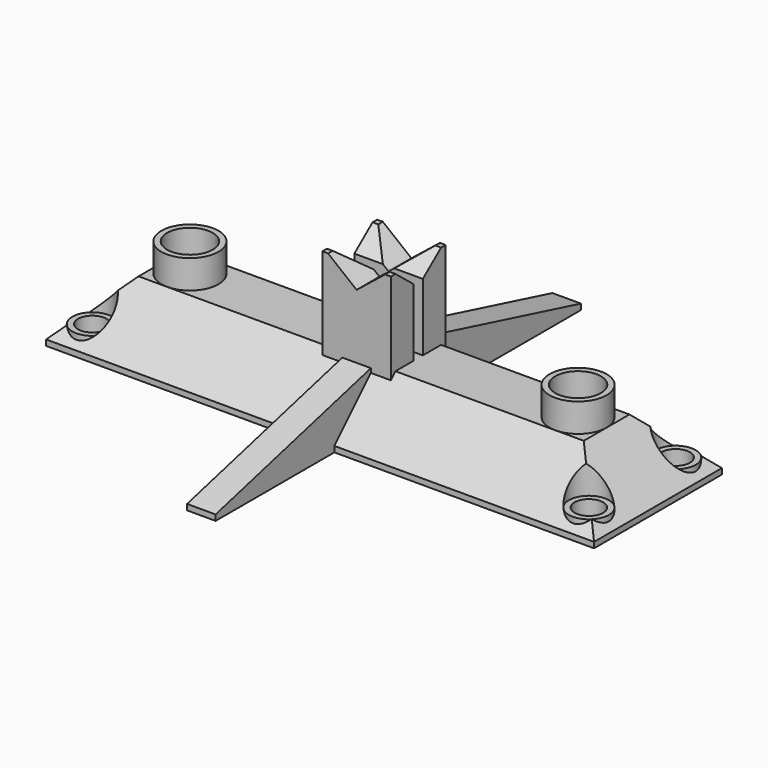
from build123d import *

# Parameters (mm, degrees)
F0_R         = 3.5
F0_R_2       = 5
F0_W         = 5
F0_H         = 26
F0_W_2       = 2.5
F0_H_2       = 6
F0_W_3       = 3.5
F1_DEPTH     = 10
F0_R_3       = 4
F2_DEPTH     = 15
F3_DEPTH     = 1
F4_T4_DEPTH  = 74.2902937834
F4_S5_R      = 5
F4_T6_DEPTH  = 39
F4_T10_DEPTH = 74.2902937834
F4_S11_R     = 5
F4_T12_DEPTH = 39
F4_T16_DEPTH = 91.7902937834
F4_T21_DEPTH = 68.6451468917
F4_S22_R     = 5
F4_T23_DEPTH = 36
F4_T27_DEPTH = 68.6451468917
F4_S28_R     = 5
F4_T29_DEPTH = 36
F4_T33_DEPTH = 91.7902937834
F4_T38_DEPTH = 91.7902937834
F4_T43_DEPTH = 68.6451468917
F4_S44_R     = 5
F4_T45_DEPTH = 36
F4_T49_DEPTH = 68.6451468917
F4_S50_R     = 5
F4_T51_DEPTH = 36
F4_T55_DEPTH = 91.7902937834
F5_SIZE2     = 9
F5_SIZE      = 35
F0_R_4       = 2.5
F6_DEPTH     = 3
F7_DEPTH     = 25
F8_W         = 2
F8_H         = 7
F10_DEPTH    = 25
F11_DEPTH    = 25


# Not quite as in the source:
# - a fillet or chamfer that OpenCascade refuses, or shapes differently, is made with other operations: its cross-section is extruded or revolved along the edge and cut away or added


with BuildPart() as f1:
    # F0 (on Top) → F1 (new body)
    with BuildSketch(Plane.XY):
        Polygon((-2.5, 14), (-48, 14), (-48, -14), (-2.5, -14), (-2.5, -6), (-6, -6), (-6, 0), (-6, 6), (-2.5, 6), align=None)
        with Locations((-43.5, -9.5)):
            Circle(F0_R, mode=Mode.SUBTRACT)
        with Locations((-43.5, 9.5)):
            Circle(F0_R, mode=Mode.SUBTRACT)
        with Locations((-34, 0)):
            Circle(F0_R_2, mode=Mode.SUBTRACT)
        Polygon((48, 14), (2.5, 14), (2.5, 6), (6, 6), (6, 0), (6, -6), (2.5, -6), (2.5, -14), (48, -14), align=None)
        with Locations((43.5, -9.5)):
            Circle(F0_R, mode=Mode.SUBTRACT)
        with Locations((34, 0)):
            Circle(F0_R_2, mode=Mode.SUBTRACT)
        with Locations((43.5, 9.5)):
            Circle(F0_R, mode=Mode.SUBTRACT)
        Polygon((-2.5, -6), (-2.5, -14), (2.5, -14), (2.5, -6), (0, -6), align=None)
        with Locations((0, -27)):
            Rectangle(F0_W, F0_H)
        Polygon((2.5, 14), (-2.5, 14), (-2.5, 6), (0, 6), (2.5, 6), align=None)
        with Locations((0, 27)):
            Rectangle(F0_W, F0_H)
        with Locations((1.25, -3)):
            Rectangle(F0_W_2, F0_H_2)
        with Locations((4.25, -3)):
            Rectangle(F0_W_3, F0_H_2)
        with Locations((-4.25, -3)):
            Rectangle(F0_W_3, F0_H_2)
        with Locations((-1.25, -3)):
            Rectangle(F0_W_2, F0_H_2)
        with Locations((-1.25, 3)):
            Rectangle(F0_W_2, F0_H_2)
        with Locations((-4.25, 3)):
            Rectangle(F0_W_3, F0_H_2)
        with Locations((4.25, 3)):
            Rectangle(F0_W_3, F0_H_2)
        with Locations((1.25, 3)):
            Rectangle(F0_W_2, F0_H_2)
    extrude(amount=F1_DEPTH)

    # F0 (on Top) → F2 (join)
    with BuildSketch(Plane.XY):
        with Locations((-34, 0)):
            Circle(F0_R_2)
        with Locations((-34, 0)):
            Circle(F0_R_3, mode=Mode.SUBTRACT)
        with Locations((34, 0)):
            Circle(F0_R_2)
        with Locations((34, 0)):
            Circle(F0_R_3, mode=Mode.SUBTRACT)
    extrude(amount=F2_DEPTH)

    # F0 (on Top) → F3 (join)
    with BuildSketch(Plane.XY):
        with Locations((-34, 0)):
            Circle(F0_R_3)
        with Locations((34, 0)):
            Circle(F0_R_3)
    extrude(amount=F3_DEPTH)

    # F4: chamfer of 9 on 6 edges, made by hand


with BuildPart() as f4_tool2:
    # F4_s3 → F4_t4 (new body)
    with BuildSketch(Plane.XZ.offset(37.1451468917)):
        Polygon((39, 10), (48, 1), (48, 10), align=None)
    extrude(amount=-F4_T4_DEPTH)

    # F4_s5 → F4_t6 (cut, symmetric)
    with BuildSketch(Plane.XY.offset(5.5)):
        with Locations((34, 0)):
            Circle(F4_S5_R)
    extrude(amount=F4_T6_DEPTH, both=True, mode=Mode.SUBTRACT)


with BuildPart() as f1_1:
    add(f1.part)

    # F4_t1: cut F4_tool2
    add(f4_tool2.part, mode=Mode.SUBTRACT)


with BuildPart() as f4_tool8:
    # F4_s9 → F4_t10 (new body)
    with BuildSketch(Plane.XZ.offset(-37.1451468917)):
        Polygon((-48, 1), (-39, 10), (-48, 10), align=None)
    extrude(amount=F4_T10_DEPTH)

    # F4_s11 → F4_t12 (cut, symmetric)
    with BuildSketch(Plane.XY.offset(5.5)):
        with Locations((-34, 0)):
            Circle(F4_S11_R)
    extrude(amount=F4_T12_DEPTH, both=True, mode=Mode.SUBTRACT)


with BuildPart() as f1_2:
    add(f1_1.part)

    # F4_t7: cut F4_tool8
    add(f4_tool8.part, mode=Mode.SUBTRACT)


with BuildPart() as f4_tool14:
    # F4_s15 → F4_t16 (new body)
    with BuildSketch(Plane.YZ.offset(20.6451468917)):
        Polygon((14, 1), (5, 10), (14, 10), align=None)
    extrude(amount=-F4_T16_DEPTH)

    split(bisect_by=Plane.YZ.offset(2.5), keep=Keep.TOP)


with BuildPart() as f1_3:
    add(f1_2.part)

    # F4_t13: cut F4_tool14
    add(f4_tool14.part, mode=Mode.SUBTRACT)


with BuildPart() as f4_tool19:
    # F4_s20 → F4_t21 (new body)
    with BuildSketch(Plane.YZ.offset(-2.5)):
        Polygon((14, 1), (5, 10), (14, 10), align=None)
    extrude(amount=-F4_T21_DEPTH)

    # F4_s22 → F4_t23 (cut, symmetric)
    with BuildSketch(Plane.XY.offset(5.5)):
        with Locations((-34, 0)):
            Circle(F4_S22_R)
    extrude(amount=F4_T23_DEPTH, both=True, mode=Mode.SUBTRACT)


with BuildPart() as f1_4:
    add(f1_3.part)

    # F4_t18: cut F4_tool19
    add(f4_tool19.part, mode=Mode.SUBTRACT)


with BuildPart() as f4_tool25:
    # F4_s26 → F4_t27 (new body)
    with BuildSketch(Plane.YZ.offset(71.1451468917)):
        Polygon((5, 10), (14, 1), (14, 10), align=None)
    extrude(amount=-F4_T27_DEPTH)

    # F4_s28 → F4_t29 (cut, symmetric)
    with BuildSketch(Plane.XY.offset(5.5)):
        with Locations((34, 0)):
            Circle(F4_S28_R)
    extrude(amount=F4_T29_DEPTH, both=True, mode=Mode.SUBTRACT)


with BuildPart() as f1_5:
    add(f1_4.part)

    # F4_t24: cut F4_tool25
    add(f4_tool25.part, mode=Mode.SUBTRACT)


with BuildPart() as f4_tool31:
    # F4_s32 → F4_t33 (new body)
    with BuildSketch(Plane.YZ.offset(71.1451468917)):
        Polygon((5, 10), (14, 1), (14, 10), align=None)
    extrude(amount=-F4_T33_DEPTH)

    split(bisect_by=Plane.YZ.offset(-2.5), keep=Keep.BOTTOM)


with BuildPart() as f1_6:
    add(f1_5.part)

    # F4_t30: cut F4_tool31
    add(f4_tool31.part, mode=Mode.SUBTRACT)


with BuildPart() as f4_tool36:
    # F4_s37 → F4_t38 (new body)
    with BuildSketch(Plane.YZ.offset(-20.6451468917)):
        Polygon((-5, 10), (-14, 1), (-14, 10), align=None)
    extrude(amount=F4_T38_DEPTH)

    split(bisect_by=Plane.YZ.offset(-2.5), keep=Keep.BOTTOM)


with BuildPart() as f1_7:
    add(f1_6.part)

    # F4_t35: cut F4_tool36
    add(f4_tool36.part, mode=Mode.SUBTRACT)


with BuildPart() as f4_tool41:
    # F4_s42 → F4_t43 (new body)
    with BuildSketch(Plane.YZ.offset(2.5)):
        Polygon((-5, 10), (-14, 1), (-14, 10), align=None)
    extrude(amount=F4_T43_DEPTH)

    # F4_s44 → F4_t45 (cut, symmetric)
    with BuildSketch(Plane.XY.offset(5.5)):
        with Locations((34, 0)):
            Circle(F4_S44_R)
    extrude(amount=F4_T45_DEPTH, both=True, mode=Mode.SUBTRACT)


with BuildPart() as f1_8:
    add(f1_7.part)

    # F4_t40: cut F4_tool41
    add(f4_tool41.part, mode=Mode.SUBTRACT)


with BuildPart() as f4_tool47:
    # F4_s48 → F4_t49 (new body)
    with BuildSketch(Plane.YZ.offset(-71.1451468917)):
        Polygon((-14, 1), (-5, 10), (-14, 10), align=None)
    extrude(amount=F4_T49_DEPTH)

    # F4_s50 → F4_t51 (cut, symmetric)
    with BuildSketch(Plane.XY.offset(5.5)):
        with Locations((-34, 0)):
            Circle(F4_S50_R)
    extrude(amount=F4_T51_DEPTH, both=True, mode=Mode.SUBTRACT)


with BuildPart() as f1_9:
    add(f1_8.part)

    # F4_t46: cut F4_tool47
    add(f4_tool47.part, mode=Mode.SUBTRACT)


with BuildPart() as f4_tool53:
    # F4_s54 → F4_t55 (new body)
    with BuildSketch(Plane.YZ.offset(-71.1451468917)):
        Polygon((-14, 1), (-5, 10), (-14, 10), align=None)
    extrude(amount=F4_T55_DEPTH)

    split(bisect_by=Plane.YZ.offset(2.5), keep=Keep.TOP)


with BuildPart() as f1_10:
    add(f1_9.part)

    # F4_t52: cut F4_tool53
    add(f4_tool53.part, mode=Mode.SUBTRACT)

    # F5
    f5_edges = [f1_10.edges().sort_by_distance(p)[0] for p in [
        (0, 40, 10),
        (0, -40, 10),
    ]]
    f5_side = f1_10.faces().sort_by_distance((0, 0, 10))[0]
    chamfer(f5_edges, length=F5_SIZE, length2=F5_SIZE2, reference=f5_side)

    # F0 (on Top) → F6 (join)
    with BuildSketch(Plane.XY):
        with Locations((-43.5, -9.5)):
            Circle(F0_R)
        with Locations((-43.5, -9.5)):
            Circle(F0_R_4, mode=Mode.SUBTRACT)
        with Locations((-43.5, 9.5)):
            Circle(F0_R)
        with Locations((-43.5, 9.5)):
            Circle(F0_R_4, mode=Mode.SUBTRACT)
        with Locations((43.5, 9.5)):
            Circle(F0_R)
        with Locations((43.5, 9.5)):
            Circle(F0_R_4, mode=Mode.SUBTRACT)
        with Locations((43.5, -9.5)):
            Circle(F0_R)
        with Locations((43.5, -9.5)):
            Circle(F0_R_4, mode=Mode.SUBTRACT)
    extrude(amount=F6_DEPTH)

    # F0 (on Top) → F7 (join)
    with BuildSketch(Plane.XY):
        with Locations((4.25, -3)):
            Rectangle(F0_W_3, F0_H_2)
        with Locations((1.25, -3)):
            Rectangle(F0_W_2, F0_H_2)
        with Locations((-1.25, -3)):
            Rectangle(F0_W_2, F0_H_2)
        with Locations((-4.25, -3)):
            Rectangle(F0_W_3, F0_H_2)
        with Locations((-4.25, 3)):
            Rectangle(F0_W_3, F0_H_2)
        with Locations((-1.25, 3)):
            Rectangle(F0_W_2, F0_H_2)
        with Locations((4.25, 3)):
            Rectangle(F0_W_3, F0_H_2)
        with Locations((1.25, 3)):
            Rectangle(F0_W_2, F0_H_2)
    extrude(amount=F7_DEPTH)

    # F8 (on face) → F10 (cut)
    with BuildSketch(Plane.YZ.offset(6)):
        Polygon((-1, 25), (-5, 25), (-1, 21.8), align=None)
        Polygon((-1, 25), (-1, 21.8), (0, 21), (1, 21.8), (1, 25), align=None)
        Polygon((5, 25), (1, 25), (1, 21.8), align=None)
        Polygon((0, 21), (-1, 21.8), (-1, 17), (1, 17), (1, 21.8), align=None)
        with Locations((0, 13.5)):
            Rectangle(F8_W, F8_H)
    extrude(amount=-F10_DEPTH, mode=Mode.SUBTRACT)

    # F9 (on face) → F11 (cut)
    with BuildSketch(Plane.XZ.offset(6)):
        Polygon((-1, 25), (-1, 21.8), (0, 21), (1, 21.8), (1, 25), align=None)
        Polygon((-1, 25), (-5, 25), (-1, 21.8), align=None)
        Polygon((5, 25), (1, 25), (1, 21.8), align=None)
    extrude(amount=-F11_DEPTH, mode=Mode.SUBTRACT)


solid = f1_10.part
